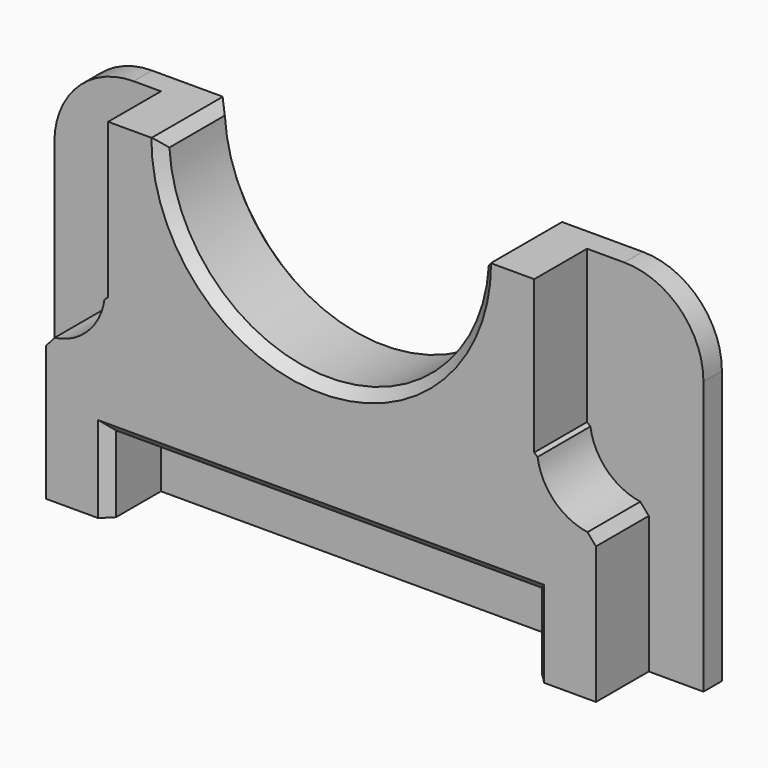
from build123d import *

# Parameters (mm, degrees)
F0_W         = 124.8875334859
F0_H         = 67.7581354976
F1_DEPTH     = 4.445
F2_R         = 15.24
F4_DEPTH     = 12.7
F6_DEPTH     = 50.8
F8_DEPTH     = 12.7
F9_T1_DEPTH  = 26.6729642247
F9_T3_DEPTH  = 19.5947973283
F9_T5_DEPTH  = 81.9930359721
F9_T7_DEPTH  = 17.2644261819
F9_T10_ANGLE = 198.2651986278
F9_T12_ANGLE = 198.2651986278
F9_T16_DEPTH = 17.2644261819
F9_T21_DEPTH = 17.2644261819
F9_T27_DEPTH = 86.8920920642
F9_T31_DEPTH = 19.5947973283
F9_T38_DEPTH = 19.5947973283
F9_T42_DEPTH = 86.8920920642


# Not quite as in the source:
# - a fillet or chamfer that OpenCascade refuses, or shapes differently, is made with other operations: its cross-section is extruded or revolved along the edge and cut away or added


with BuildPart() as f1:
    # F0 (on Front) → F1 (new body)
    with BuildSketch(Plane.XZ):
        with Locations((0.9489916265, 33.8790677488)):
            Rectangle(F0_W, F0_H)
    extrude(amount=F1_DEPTH)

    # F2
    f2_edges = [f1.edges().sort_by_distance(p)[0] for p in [
        (-61.494775, -2.2225, 67.758135),
        (63.392758, -2.2225, 67.758135),
    ]]
    fillet(f2_edges, radius=F2_R)

    # F3 (on face) → F4 (join)
    with BuildSketch(Plane.XZ.offset(4.445)):
        Polygon((40.9965217113, 67.7581354976), (-40.9965142608, 67.7581354976), (-40.9965142608, 39.0565320849), (-40.9965142608, 14.6957412362), (40.9965217113, 14.6957412362), (40.9965217113, 39.4814237952), align=None)
        Polygon((-40.9965142608, 14.6957412362), (-40.9965142608, 39.0565320849), (-52.9372058809, 39.0565320849), (-52.9372058809, 0), (-40.9965142608, 0), align=None)
        Polygon((52.8750233352, 39.4814237952), (40.9965217113, 39.4814237952), (40.9965217113, 14.6957412362), (40.9965217113, 0), (52.8750233352, 0), align=None)
    extrude(amount=F4_DEPTH)

    # F5 (on face) → F6 (cut)
    with BuildSketch(Plane.XZ.offset(17.145)):
        with BuildLine():
            ThreePointArc((-30.7849538809, 67.7581354976), (0, 36.9731816167), (30.7849538809, 67.7581354976))
            Line((30.7849538809, 67.7581354976), (-30.7849538809, 67.7581354976))
        make_face()
        with BuildLine():
            Line((-30.7849538809, 67.7581354976), (30.7849538809, 67.7581354976))
            ThreePointArc((30.7849538809, 67.7581354976), (0, 98.5430893784), (-30.7849538809, 67.7581354976))
        make_face()
    extrude(amount=-F6_DEPTH, mode=Mode.SUBTRACT)

    # F7 (on face) → F8 (cut)
    with BuildSketch(Plane.XZ.offset(17.145)):
        with BuildLine():
            ThreePointArc((-52.9372058809, 27.6993892785), (-44.9064931875, 31.0258193916), (-41.5800630744, 39.0565320849))
            Line((-41.5800630744, 39.0565320849), (-52.9372058809, 39.0565320849))
            Line((-52.9372058809, 39.0565320849), (-52.9372058809, 27.6993892785))
        make_face()
        with BuildLine():
            Line((52.8750233352, 39.4814237952), (41.5178805288, 39.4814237952))
            ThreePointArc((41.5178805288, 39.4814237952), (44.8443106419, 31.4507111019), (52.8750233352, 28.1242809888))
            Line((52.8750233352, 28.1242809888), (52.8750233352, 39.4814237952))
        make_face()
    extrude(amount=-F8_DEPTH, mode=Mode.SUBTRACT)

    # F9: chamfer of 1.905 on 11 edges, made by hand

    # F9_s2 → F9_t1 (cut)
    with BuildSketch(Plane.XZ.offset(-4.7639821123)):
        with BuildLine():
            Line((-32.6343999444, 67.7581354976), (-30.7326373381, 65.964148961))
            ThreePointArc((-30.7326373381, 65.964148961), (-30.7710738122, 66.8337968736), (-30.7849538809, 67.7581354976))
            Line((-30.7849538809, 67.7581354976), (-32.6343999444, 67.7581354976))
        make_face()
        with BuildLine():
            Line((30.7326373381, 65.964148961), (32.6343999444, 67.7581354976))
            Line((32.6343999444, 67.7581354976), (30.7849538809, 67.7581354976))
            ThreePointArc((30.7849538809, 67.7581354976), (30.7710738122, 66.8337968736), (30.7326373381, 65.964148961))
        make_face()
    extrude(amount=F9_T1_DEPTH, mode=Mode.SUBTRACT)

    # F9_s4 → F9_t3 (cut)
    with BuildSketch(Plane.XY.offset(-4.8990560921)):
        Polygon((-42.9015142608, -17.145), (-40.9965142608, -15.24), (-40.9965142608, -17.145), align=None)
        Polygon((42.9015217113, -17.145), (40.9965217113, -15.24), (40.9965217113, -17.145), align=None)
    extrude(amount=F9_T3_DEPTH, mode=Mode.SUBTRACT)

    # F9_s6 → F9_t5 (cut)
    with BuildSketch(Plane.YZ.offset(-40.9965142608)):
        Polygon((-17.145, 16.6007412362), (-15.24, 14.6957412362), (-17.145, 14.6957412362), align=None)
    extrude(amount=F9_T5_DEPTH, mode=Mode.SUBTRACT)

    # F9_s8 → F9_t7 (cut)
    with BuildSketch(Plane.XZ.offset(4.445)):
        with BuildLine():
            Line((52.8750233352, 26.356813065), (51.2436612422, 28.24205769))
            ThreePointArc((51.2436612422, 28.24205769), (52.0302167258, 28.1557452496), (52.8750233352, 28.1242809888))
            Line((52.8750233352, 28.1242809888), (52.8750233352, 26.356813065))
        make_face()
        with BuildLine():
            Line((-52.9372058809, 25.9319213547), (-51.3058437879, 27.8171659797))
            ThreePointArc((-51.3058437879, 27.8171659797), (-52.0923992715, 27.7308535393), (-52.9372058809, 27.6993892785))
            Line((-52.9372058809, 27.6993892785), (-52.9372058809, 25.9319213547))
        make_face()
    extrude(amount=F9_T7_DEPTH, mode=Mode.SUBTRACT)

    # F9_s9 → F9_t10 (revolve, cut)
    with BuildSketch(Plane(origin=(10.6182323587, 0, 66.0511732612), x_dir=(0, 1, 0), z_dir=(0.1587198459, 0, 0.9873236605))):
        Polygon((-15.24, 41.539514704), (-17.145, 43.444514704), (-17.145, 41.539514704), align=None)
    revolve(axis=Axis((0, -17.145, 67.7581354976), (0, -1, 0)), revolution_arc=F9_T10_ANGLE, mode=Mode.SUBTRACT)

    # F9_s11 → F9_t12 (revolve, cut)
    with BuildSketch(Plane(origin=(10.6182323587, 0, 66.0511732612), x_dir=(0, 1, 0), z_dir=(0.1587198459, 0, 0.9873236605))):
        Polygon((0, 43.444514704), (-1.905, 41.539514704), (0, 41.539514704), align=None)
    revolve(axis=Axis((0, 0, 67.7581354976), (0, -1, 0)), revolution_arc=F9_T12_ANGLE, mode=Mode.SUBTRACT)


with BuildPart() as f9_tool14:
    # F9_s15 → F9_t16 (new body)
    with BuildSketch(Plane.XZ.offset(21.7094261819)):
        with BuildLine():
            Line((41.63565723, 37.8500617022), (39.750412605, 39.4814237952))
            Line((39.750412605, 39.4814237952), (41.5178805288, 39.4814237952))
            ThreePointArc((41.5178805288, 39.4814237952), (41.5493447896, 38.6366171858), (41.63565723, 37.8500617022))
        make_face()
    extrude(amount=-F9_T16_DEPTH)

    split(bisect_by=Plane.YZ.offset(40.9965217113), keep=Keep.TOP)


with BuildPart() as f1_1:
    add(f1.part)

    # F9_t13: cut F9_tool14
    add(f9_tool14.part, mode=Mode.SUBTRACT)


with BuildPart() as f9_tool19:
    # F9_s20 → F9_t21 (new body)
    with BuildSketch(Plane.XZ.offset(21.7094261819)):
        with BuildLine():
            Line((-39.8125951507, 39.0565320849), (-41.6978397756, 37.4251699919))
            ThreePointArc((-41.6978397756, 37.4251699919), (-41.6115273352, 38.2117254755), (-41.5800630744, 39.0565320849))
            Line((-41.5800630744, 39.0565320849), (-39.8125951507, 39.0565320849))
        make_face()
    extrude(amount=-F9_T21_DEPTH)

    split(bisect_by=Plane.YZ.offset(-40.9965142608), keep=Keep.BOTTOM)


with BuildPart() as f1_2:
    add(f1_1.part)

    # F9_t18: cut F9_tool19
    add(f9_tool19.part, mode=Mode.SUBTRACT)


with BuildPart() as f9_tool25:
    # F9_s26 → F9_t27 (new body)
    with BuildSketch(Plane.YZ.offset(-45.8955703528)):
        Polygon((-17.145, 16.6007412362), (-15.24, 14.6957412362), (-17.145, 14.6957412362), align=None)
    extrude(amount=F9_T27_DEPTH)

    split(bisect_by=Plane.YZ.offset(-40.9965142608), keep=Keep.BOTTOM)


with BuildPart() as f9_tool29:
    # F9_s30 → F9_t31 (new body)
    with BuildSketch(Plane.XY):
        Polygon((-42.9015142608, -17.145), (-40.9965142608, -15.24), (-40.9965142608, -17.145), align=None)
    extrude(amount=F9_T31_DEPTH)

    split(bisect_by=Plane.XY.offset(14.6957412362), keep=Keep.TOP)


with BuildPart() as f9_tool25_1:
    add(f9_tool25.part)

    # F9_t33: intersect F9_tool29
    add(f9_tool29.part, mode=Mode.INTERSECT)


with BuildPart() as f1_3:
    add(f1_2.part)

    # F9_t23: cut F9_tool25
    add(f9_tool25_1.part, mode=Mode.SUBTRACT)


with BuildPart() as f9_tool36:
    # F9_s37 → F9_t38 (new body)
    with BuildSketch(Plane.XY.offset(19.5947973283)):
        Polygon((42.9015217113, -17.145), (40.9965217113, -15.24), (40.9965217113, -17.145), align=None)
    extrude(amount=-F9_T38_DEPTH)

    split(bisect_by=Plane.XY.offset(14.6957412362), keep=Keep.TOP)


with BuildPart() as f9_tool40:
    # F9_s41 → F9_t42 (new body)
    with BuildSketch(Plane.YZ.offset(-40.9965142608)):
        Polygon((-17.145, 16.6007412362), (-15.24, 14.6957412362), (-17.145, 14.6957412362), align=None)
    extrude(amount=F9_T42_DEPTH)

    split(bisect_by=Plane.YZ.offset(40.9965217113), keep=Keep.TOP)


with BuildPart() as f9_tool36_1:
    add(f9_tool36.part)

    # F9_t44: intersect F9_tool40
    add(f9_tool40.part, mode=Mode.INTERSECT)


with BuildPart() as f1_4:
    add(f1_3.part)

    # F9_t34: cut F9_tool36
    add(f9_tool36_1.part, mode=Mode.SUBTRACT)


solid = f1_4.part
